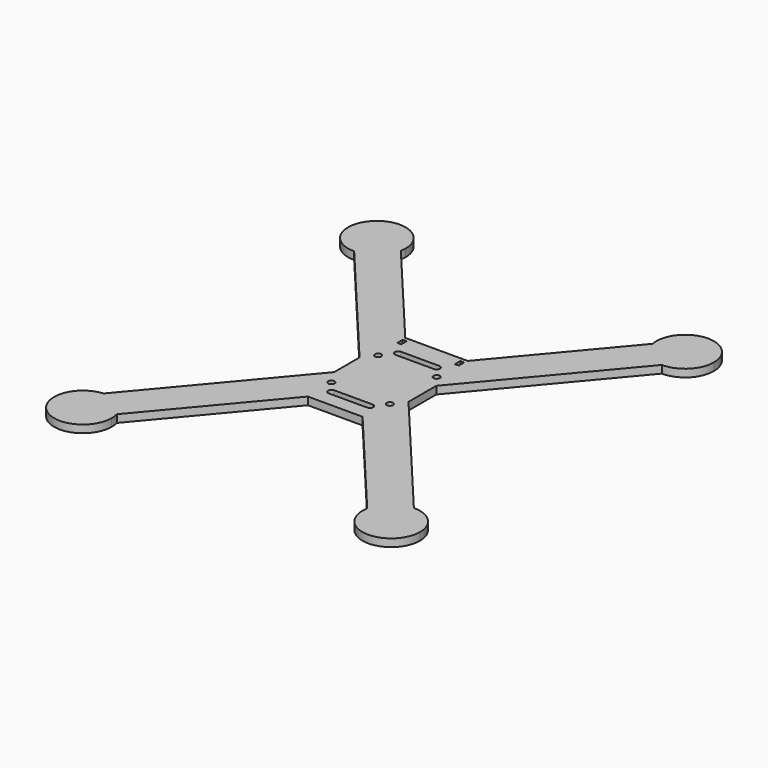
from build123d import *

# Parameters (mm, degrees)
F0_R     = 1.65
F1_DEPTH = 4


with BuildPart() as f1:
    # F0 (on Top) → F1 (new body)
    with BuildSketch(Plane.XY):
        with BuildLine():
            Line((-20, 34.1743044555), (-20, 20))
            Line((-20, 20), (-20, 9.0556954967))
            Line((-20, 9.0556954967), (-20, -7.4999716698))
            Line((-20, -7.4999716698), (-20, -20))
            Line((-20, -20), (-20, -31))
            Line((-20, -31), (-14.9161266072, -31))
            Line((-14.9161266072, -31), (-8.6228793733, -23.5))
            Line((-8.6228793733, -23.5), (-10, -23.5))
            ThreePointArc((-10, -23.5), (-11.75, -21.75), (-10, -20))
            Line((-10, -20), (-5.6860306642, -20))
            Line((-5.6860306642, -20), (4.3806233749, -20))
            Line((4.3806233749, -20), (10, -20))
            ThreePointArc((10, -20), (11.2374368671, -20.5125631329), (11.75, -21.75))
            ThreePointArc((11.75, -21.75), (11.2374368671, -22.9874368671), (10, -23.5))
            Line((10, -23.5), (7.317472084, -23.5))
            Line((7.317472084, -23.5), (13.6107193178, -31))
            Line((13.6107193178, -31), (20, -31))
            Line((20, -31), (20, -20))
            Line((20, -20), (20, -9.0556954967))
            Line((20, -9.0556954967), (20, 9.0556954967))
            Line((20, 9.0556954967), (20, 20))
            Line((20, 20), (20, 34.1743044555))
            Line((20, 34.1743044555), (16.2742770157, 34.1743044555))
            Line((16.2742770157, 34.1743044555), (14.5960777534, 32.1743044555))
            Line((14.5960777534, 32.1743044555), (16, 32.1743044555))
            Line((16, 32.1743044555), (16, 28.6743044555))
            Line((16, 28.6743044555), (14, 28.6743044555))
            Line((14, 28.6743044555), (14, 31.4639266515))
            Line((14, 31.4639266515), (7.317472084, 23.5))
            Line((7.317472084, 23.5), (10, 23.5))
            ThreePointArc((10, 23.5), (11.2374368671, 22.9874368671), (11.75, 21.75))
            ThreePointArc((11.75, 21.75), (11.2374368671, 20.5125631329), (10, 20))
            Line((10, 20), (0, 20))
            Line((0, 20), (-4.3806233749, 20))
            Line((-4.3806233749, 20), (-10, 20))
            ThreePointArc((-10, 20), (-11.75, 21.75), (-10, 23.5))
            Line((-10, 23.5), (-7.317472084, 23.5))
            Line((-7.317472084, 23.5), (-14, 31.4639266515))
            Line((-14, 31.4639266515), (-14, 28.6743044555))
            Line((-14, 28.6743044555), (-16, 28.6743044555))
            Line((-16, 28.6743044555), (-16, 32.1743044555))
            Line((-16, 32.1743044555), (-14.5960777534, 32.1743044555))
            Line((-14.5960777534, 32.1743044555), (-16.2742770157, 34.1743044555))
            Line((-16.2742770157, 34.1743044555), (-20, 34.1743044555))
        make_face()
        with Locations((-15.25, -15.25)):
            Circle(F0_R, mode=Mode.SUBTRACT)
        with Locations((15.25, -15.25)):
            Circle(F0_R, mode=Mode.SUBTRACT)
        with Locations((-15.25, 15.25)):
            Circle(F0_R, mode=Mode.SUBTRACT)
        with Locations((15.25, 15.25)):
            Circle(F0_R, mode=Mode.SUBTRACT)
        with BuildLine():
            Line((-20, 9.0556954967), (-20, 20))
            Line((-20, 20), (-20, 34.1743044555))
            Line((-20, 34.1743044555), (-16.2742770157, 34.1743044555))
            Line((-16.2742770157, 34.1743044555), (-65.6094303769, 92.9696507149))
            ThreePointArc((-65.6094303769, 92.9696507149), (-70.7066370655, 84.2648887431), (-80.1642747962, 80.7566861309))
            Line((-80.1642747962, 80.7566861309), (-20, 9.0556954967))
        make_face()
        with BuildLine():
            Line((-20, -20), (-20, -7.4999716698))
            Line((-20, -7.4999716698), (-81.5062852996, -80.8003081427))
            ThreePointArc((-81.5062852996, -80.8003081427), (-71.7350386168, -83.4751187737), (-65.8927282585, -91.7515481563))
            Line((-65.8927282585, -91.7515481563), (-14.9161266072, -31))
            Line((-14.9161266072, -31), (-20, -31))
            Line((-20, -31), (-20, -20))
        make_face()
        with BuildLine():
            ThreePointArc((-65.3484512108, 95.7555553899), (-91.0199704611, 106.2968397941), (-80.1642747962, 80.7566861309))
            Line((-80.1642747962, 80.7566861309), (-87.6258734204, 89.6490730979))
            Line((-87.6258734204, 89.6490730979), (-80.3484512108, 95.7555553899))
            Line((-80.3484512108, 95.7555553899), (-73.0710290012, 101.8620376819))
            Line((-73.0710290012, 101.8620376819), (-65.6094303769, 92.9696507149))
            ThreePointArc((-65.6094303769, 92.9696507149), (-65.413838519, 94.3565043737), (-65.3484512108, 95.7555553899))
        make_face()
        with BuildLine():
            Line((-87.6258734204, 89.6490730979), (-80.1642747962, 80.7566861309))
            ThreePointArc((-80.1642747962, 80.7566861309), (-70.7066370655, 84.2648887431), (-65.6094303769, 92.9696507149))
            Line((-65.6094303769, 92.9696507149), (-73.0710290012, 101.8620376819))
            Line((-73.0710290012, 101.8620376819), (-80.3484512108, 95.7555553899))
            Line((-80.3484512108, 95.7555553899), (-87.6258734204, 89.6490730979))
        make_face()
        Polygon((16.2742770157, 34.1743044555), (-16.2742770157, 34.1743044555), (-14.5960777534, 32.1743044555), (-14, 32.1743044555), (-14, 31.4639266515), (-7.317472084, 23.5), (7.317472084, 23.5), (14, 31.4639266515), (14, 32.1743044555), (14.5960777534, 32.1743044555), align=None)
        with BuildLine():
            ThreePointArc((-65.8927282585, -91.7515481563), (-71.7350386168, -83.4751187737), (-81.5062852996, -80.8003081427))
            Line((-81.5062852996, -80.8003081427), (-88.3919178636, -89.0062854882))
            Line((-88.3919178636, -89.0062854882), (-80.3484512108, -95.7555553899))
            Line((-80.3484512108, -95.7555553899), (-73.8370734443, -101.2192500722))
            Line((-73.8370734443, -101.2192500722), (-65.8927282585, -91.7515481563))
        make_face()
        with BuildLine():
            Line((-88.3919178636, -89.0062854882), (-81.5062852996, -80.8003081427))
            ThreePointArc((-81.5062852996, -80.8003081427), (-90.5374768921, -106.7639047514), (-65.3484512108, -95.7555553899))
            ThreePointArc((-65.3484512108, -95.7555553899), (-65.485143297, -93.7351401212), (-65.8927282585, -91.7515481563))
            Line((-65.8927282585, -91.7515481563), (-73.8370734443, -101.2192500722))
            Line((-73.8370734443, -101.2192500722), (-80.3484512108, -95.7555553899))
            Line((-80.3484512108, -95.7555553899), (-88.3919178636, -89.0062854882))
        make_face()
        with BuildLine():
            Line((65.6094303769, 92.9696507149), (16.2742770157, 34.1743044555))
            Line((16.2742770157, 34.1743044555), (20, 34.1743044555))
            Line((20, 34.1743044555), (20, 20))
            Line((20, 20), (20, 9.0556954967))
            Line((20, 9.0556954967), (80.1642747962, 80.7566861309))
            ThreePointArc((80.1642747962, 80.7566861309), (70.7066370655, 84.2648887431), (65.6094303769, 92.9696507149))
        make_face()
        with BuildLine():
            ThreePointArc((95.3484512108, 95.7555553899), (78.9494001947, 110.6901680817), (65.6094303769, 92.9696507149))
            Line((65.6094303769, 92.9696507149), (73.0710290012, 101.8620376819))
            Line((73.0710290012, 101.8620376819), (80.3484512108, 95.7555553899))
            Line((80.3484512108, 95.7555553899), (87.6258734204, 89.6490730979))
            Line((87.6258734204, 89.6490730979), (80.1642747962, 80.7566861309))
            ThreePointArc((80.1642747962, 80.7566861309), (90.889735615, 85.0840361396), (95.3484512108, 95.7555553899))
        make_face()
        with BuildLine():
            Line((73.0710290012, 101.8620376819), (65.6094303769, 92.9696507149))
            ThreePointArc((65.6094303769, 92.9696507149), (70.7066370655, 84.2648887431), (80.1642747962, 80.7566861309))
            Line((80.1642747962, 80.7566861309), (87.6258734204, 89.6490730979))
            Line((87.6258734204, 89.6490730979), (80.3484512108, 95.7555553899))
            Line((80.3484512108, 95.7555553899), (73.0710290012, 101.8620376819))
        make_face()
        Polygon((-8.6228793733, -23.5), (-14.9161266072, -31), (13.6107193178, -31), (7.317472084, -23.5), align=None)
        with BuildLine():
            Line((20, -31), (13.6107193178, -31))
            Line((13.6107193178, -31), (65.6094303769, -92.9696507149))
            ThreePointArc((65.6094303769, -92.9696507149), (70.7066370655, -84.2648887431), (80.1642747962, -80.7566861309))
            Line((80.1642747962, -80.7566861309), (20, -9.0556954967))
            Line((20, -9.0556954967), (20, -20))
            Line((20, -20), (20, -31))
        make_face()
        with BuildLine():
            ThreePointArc((80.1642747962, -80.7566861309), (70.7066370655, -84.2648887431), (65.6094303769, -92.9696507149))
            Line((65.6094303769, -92.9696507149), (73.0710290012, -101.8620376819))
            Line((73.0710290012, -101.8620376819), (80.3484512108, -95.7555553899))
            Line((80.3484512108, -95.7555553899), (87.6258734204, -89.6490730979))
            Line((87.6258734204, -89.6490730979), (80.1642747962, -80.7566861309))
        make_face()
        with BuildLine():
            Line((73.0710290012, -101.8620376819), (65.6094303769, -92.9696507149))
            ThreePointArc((65.6094303769, -92.9696507149), (78.9494001947, -110.6901680817), (95.3484512108, -95.7555553899))
            ThreePointArc((95.3484512108, -95.7555553899), (90.889735615, -85.0840361396), (80.1642747962, -80.7566861309))
            Line((80.1642747962, -80.7566861309), (87.6258734204, -89.6490730979))
            Line((87.6258734204, -89.6490730979), (80.3484512108, -95.7555553899))
            Line((80.3484512108, -95.7555553899), (73.0710290012, -101.8620376819))
        make_face()
    extrude(amount=F1_DEPTH)


solid = f1.part
